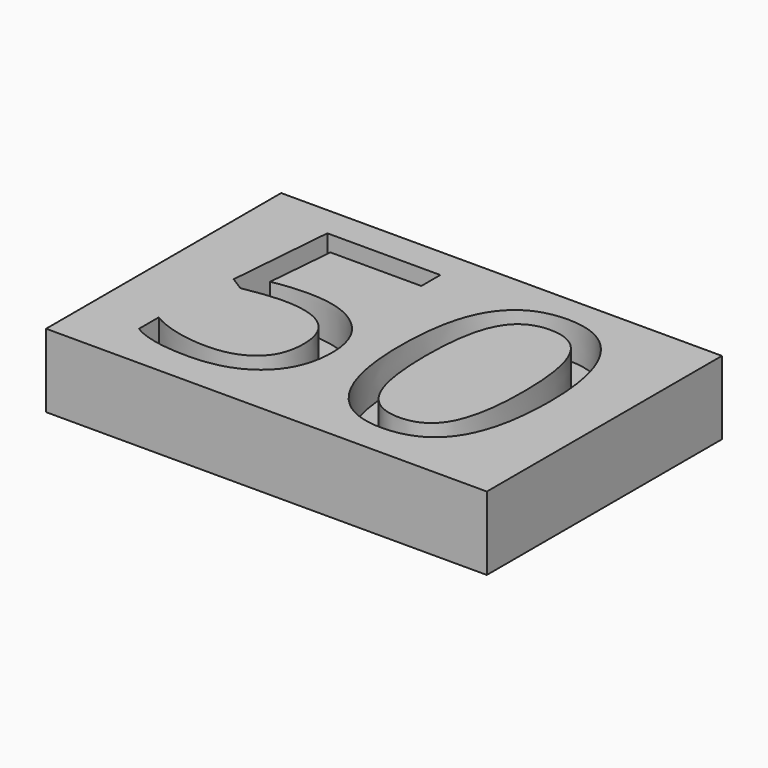
from build123d import *

# Parameters (mm, degrees)
F0_W         = 19.05
F0_H         = 12.7
F1_DEPTH     = 3.175
F2_TEXT_SIZE = 13.7567633176
F3_DEPTH     = 1.55575


# Not quite as in the source:
# - Text() gives the source's letters only with a copy of the font that has no kerning and outlines rounded to 1/6400 em; it was checked with that copy


with BuildPart() as f1:
    # F0 (on Top) → F1 (new body)
    with BuildSketch(Plane.XY):
        with Locations((9.525, 6.35)):
            Rectangle(F0_W, F0_H)
    extrude(amount=F1_DEPTH)

    # F2 (on face) → F3 (cut)
    with BuildSketch(Plane.XY.offset(3.175)):
        with Locations((1.55575, 1.55575)):
            Text('50', F2_TEXT_SIZE, font='Open Sans', text_align=(TextAlign.LEFT, TextAlign.BOTTOM))
    extrude(amount=-F3_DEPTH, mode=Mode.SUBTRACT)


solid = f1.part
